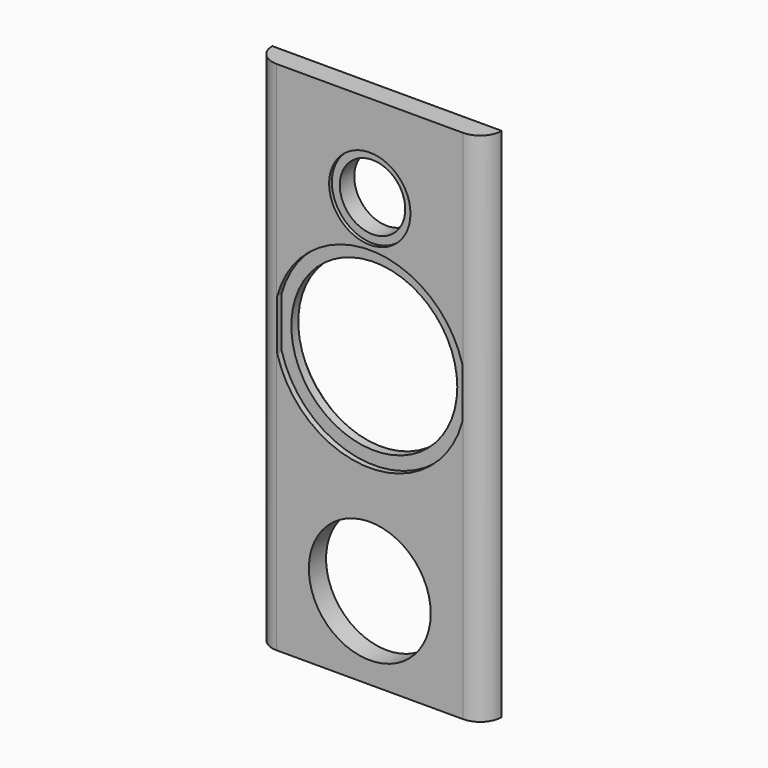
from build123d import *

# Parameters (mm, degrees)
F0_W      = 203.2
F0_H      = 457.2
F1_DEPTH  = 19.05
F2_R      = 19.04999
F3_R      = 19.04999
F5_DEPTH  = 5
F6_R      = 73.5
F7_DEPTH  = 25.4
F8_SIZE   = 6.35
F9_R      = 36
F10_DEPTH = 3
F11_R     = 29
F12_DEPTH = 25.4
F13_R     = 53.975
F14_DEPTH = 25.4


# Not quite as in the source:
# - a fillet or chamfer is up to 0.001 mm smaller than in the source, because OpenCascade refuses the exact size


with BuildPart() as f1:
    # F0 (on Front) → F1 (new body)
    with BuildSketch(Plane.XZ):
        Rectangle(F0_W, F0_H)
    extrude(amount=F1_DEPTH)

    # F2 (radius 19.05 in the source; OpenCascade refuses exactly that, so slightly less here)
    f2_edges = [f1.edges().sort_by_distance(p)[0] for p in [
        (-101.6, -19.05, 0),
    ]]
    fillet(f2_edges, radius=F2_R)

    # F3 (radius 19.05 in the source; OpenCascade refuses exactly that, so slightly less here)
    f3_edges = [f1.edges().sort_by_distance(p)[0] for p in [
        (101.6, -19.05, 0),
    ]]
    fillet(f3_edges, radius=F3_R)

    # F4 (on face) → F5 (cut)
    with BuildSketch(Plane.XZ.offset(19.05)):
        with BuildLine():
            Line((82, 3.0169707144), (82, 47.7830292856))
            ThreePointArc((82, 47.7830292856), (0, 110.4), (-82, 47.7830292856))
            Line((-82, 47.7830292856), (-82, 3.0169707144))
            ThreePointArc((-82, 3.0169707144), (0, -59.6), (82, 3.0169707144))
        make_face()
    extrude(amount=-F5_DEPTH, mode=Mode.SUBTRACT)

    # F6 (on face) → F7 (cut)
    with BuildSketch(Plane.XZ.offset(19.05)):
        with Locations((0, 25.4)):
            Circle(F6_R)
    extrude(amount=-F7_DEPTH, mode=Mode.SUBTRACT)

    # F8
    f8_edges = [f1.edges().sort_by_distance(p)[0] for p in [
        (-73.5, 0, 25.4),
    ]]
    chamfer(f8_edges, length=F8_SIZE)

    # F9 (on face) → F10 (cut)
    with BuildSketch(Plane.XZ.offset(19.05)):
        with Locations((0, 150.4)):
            Circle(F9_R)
    extrude(amount=-F10_DEPTH, mode=Mode.SUBTRACT)

    # F11 (on face) → F12 (cut)
    with BuildSketch(Plane.XZ.offset(19.05)):
        with Locations((0, 150.4)):
            Circle(F11_R)
    extrude(amount=-F12_DEPTH, mode=Mode.SUBTRACT)

    # F13 (on face) → F14 (cut)
    with BuildSketch(Plane.XZ.offset(19.05)):
        with Locations((0, -155.575)):
            Circle(F13_R)
    extrude(amount=-F14_DEPTH, mode=Mode.SUBTRACT)


solid = f1.part
